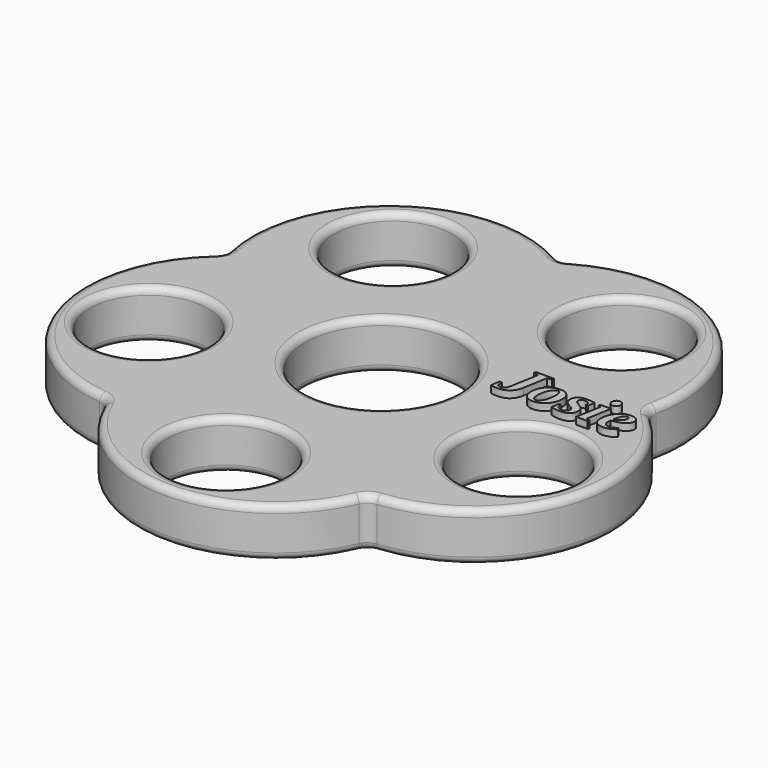
from build123d import *

# Parameters (mm, degrees)
F0_R         = 8.5
F0_R_2       = 11
F1_DEPTH     = 7
F2_R         = 2
F3_R         = 1
F4_TEXT_SIZE = 8.692171347
F5_DEPTH     = 1


# Not quite as in the source:
# - Text() gives the source's letters only with a copy of the font that has no kerning and outlines rounded to 1/6400 em; it was checked with that copy


with BuildPart() as f1:
    # F0 (on Top) → F1 (new body)
    with BuildSketch(Plane.XY):
        with BuildLine():
            ThreePointArc((30.3984422568, 9.877052624), (22.9236248394, 31.5516627806), (0, 31.9628137087))
            ThreePointArc((0, 31.9628137087), (-22.9236248394, 31.5516627806), (-30.3984422568, 9.877052624))
            ThreePointArc((-30.3984422568, 9.877052624), (-37.0912041355, -12.0516627806), (-18.7872705198, -25.8584594784))
            ThreePointArc((-18.7872705198, -25.8584594784), (0, -39), (18.7872705198, -25.8584594784))
            ThreePointArc((18.7872705198, -25.8584594784), (37.0912041355, -12.0516627806), (30.3984422568, 9.877052624))
        make_face()
        with Locations((0, -28)):
            Circle(F0_R, mode=Mode.SUBTRACT)
        with Locations((-26.6295824563, -8.6524758425)):
            Circle(F0_R, mode=Mode.SUBTRACT)
        with Locations((26.6295824563, -8.6524758425)):
            Circle(F0_R, mode=Mode.SUBTRACT)
        Circle(F0_R_2, mode=Mode.SUBTRACT)
        with Locations((-16.4579870642, 22.6524758425)):
            Circle(F0_R, mode=Mode.SUBTRACT)
        with Locations((16.4579870642, 22.6524758425)):
            Circle(F0_R, mode=Mode.SUBTRACT)
    extrude(amount=F1_DEPTH)

    # F2
    f2_edges = [f1.edges().sort_by_distance(p)[0] for p in [
        (18.787271, -25.858459, 3.5),
        (30.398442, 9.877053, 3.5),
        (0, 31.962814, 3.5),
        (-30.398442, 9.877053, 3.5),
        (-18.787271, -25.858459, 3.5),
    ]]
    fillet(f2_edges, radius=F2_R)

    # F3
    f3_edges = [f1.edges().sort_by_distance(p)[0] for p in [
        (0, -39, 7),
        (-19.000712, -26.152236, 7),
        (19.000712, -26.152236, 7),
        (-37.091204, -12.051663, 7),
        (37.091204, -12.051663, 7),
        (-30.743797, 9.989265, 7),
        (30.743797, 9.989265, 7),
        (-22.923625, 31.551663, 7),
        (22.923625, 31.551663, 7),
        (0, 32.325942, 7),
        (-8.5, -28, 7),
        (-35.129582, -8.652476, 7),
        (18.129582, -8.652476, 7),
        (-11, 0, 7),
        (-24.957987, 22.652476, 7),
        (7.957987, 22.652476, 7),
        (0, -39, 0),
        (-19.000712, -26.152236, 0),
        (19.000712, -26.152236, 0),
        (-37.091204, -12.051663, 0),
        (37.091204, -12.051663, 0),
        (-30.743797, 9.989265, 0),
        (30.743797, 9.989265, 0),
        (-22.923625, 31.551663, 0),
        (22.923625, 31.551663, 0),
        (0, 32.325942, 0),
        (-8.5, -28, 0),
        (-35.129582, -8.652476, 0),
        (18.129582, -8.652476, 0),
        (-11, 0, 0),
        (-24.957987, 22.652476, 0),
        (7.957987, 22.652476, 0),
    ]]
    fillet(f3_edges, radius=F3_R)

    # F4 (on face) → F5 (join)
    with BuildSketch(Plane.XY.offset(7)):
        with Locations((14.2256403342, 1.9055493176)):
            Text('Josie', F4_TEXT_SIZE, font='Tinos', font_style=FontStyle.BOLDITALIC, text_align=(TextAlign.LEFT, TextAlign.BOTTOM))
    extrude(amount=F5_DEPTH)


solid = f1.part
